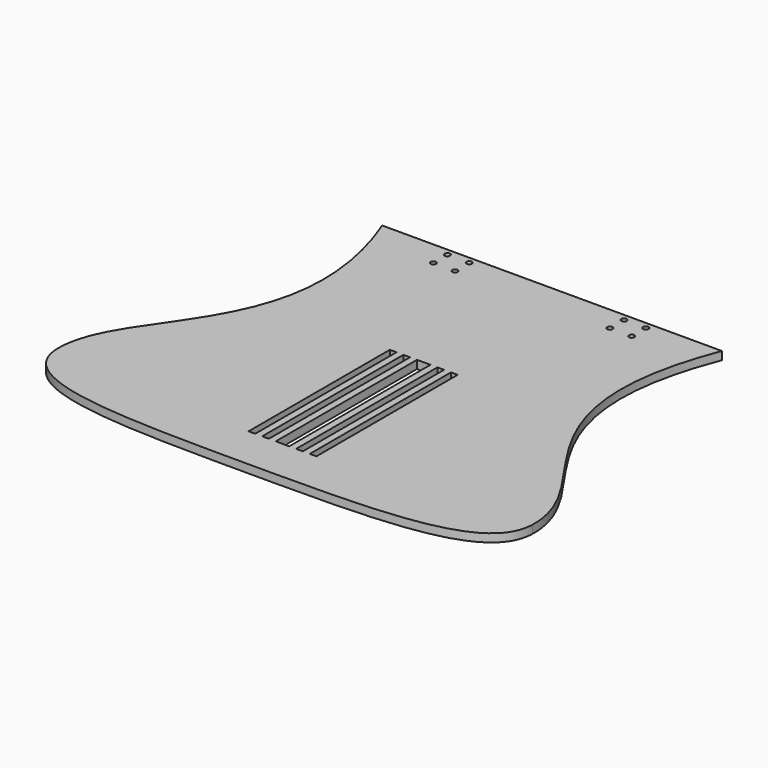
from build123d import *

# Parameters (mm, degrees)
F1_W     = 4.9
F1_H     = 129.9
F1_W_2   = 9.9
F1_R     = 2.025
F2_DEPTH = 6


with BuildPart() as f2:
    # F1 (on Top) → F2 (new body)
    with BuildSketch(Plane.XY):
        with BuildLine():
            Line((125, 0), (-125, 0))
            add(Edge.make_bspline(
                [(-125, 0), (-70.472038, -139.68512), (-176.99485, -172.72353), (-175, -236.876854)],
                knots=[0, 0, 0, 0, 1, 1, 1, 1], degree=3))
            add(Edge.make_bspline(
                [(-175, -236.876854), (-173.659084, -280), (-96.910591, -280), (0, -280)],
                knots=[0, 0, 0, 0, 1, 1, 1, 1], degree=3))
            add(Edge.make_bspline(
                [(175, -236.876854), (173.659084, -280), (96.910591, -280), (0, -280)],
                knots=[0, 0, 0, 0, 1, 1, 1, 1], degree=3))
            add(Edge.make_bspline(
                [(125, 0), (70.472038, -139.68512), (176.99485, -172.72353), (175, -236.876854)],
                knots=[0, 0, 0, 0, 1, 1, 1, 1], degree=3))
        make_face()
        with Locations((-22.5, -183)):
            Rectangle(F1_W, F1_H, mode=Mode.SUBTRACT)
        with Locations((-12.5, -183)):
            Rectangle(F1_W, F1_H, mode=Mode.SUBTRACT)
        with Locations((0, -183)):
            Rectangle(F1_W_2, F1_H, mode=Mode.SUBTRACT)
        with Locations((12.5, -183)):
            Rectangle(F1_W, F1_H, mode=Mode.SUBTRACT)
        with Locations((22.5, -183)):
            Rectangle(F1_W, F1_H, mode=Mode.SUBTRACT)
        with Locations((-73, -18)):
            Circle(F1_R, mode=Mode.SUBTRACT)
        with Locations((-57, -18)):
            Circle(F1_R, mode=Mode.SUBTRACT)
        with Locations((-73, -5)):
            Circle(F1_R, mode=Mode.SUBTRACT)
        with Locations((-57, -5)):
            Circle(F1_R, mode=Mode.SUBTRACT)
        with Locations((57, -18)):
            Circle(F1_R, mode=Mode.SUBTRACT)
        with Locations((73, -18)):
            Circle(F1_R, mode=Mode.SUBTRACT)
        with Locations((57, -5)):
            Circle(F1_R, mode=Mode.SUBTRACT)
        with Locations((73, -5)):
            Circle(F1_R, mode=Mode.SUBTRACT)
    extrude(amount=F2_DEPTH)


solid = f2.part
